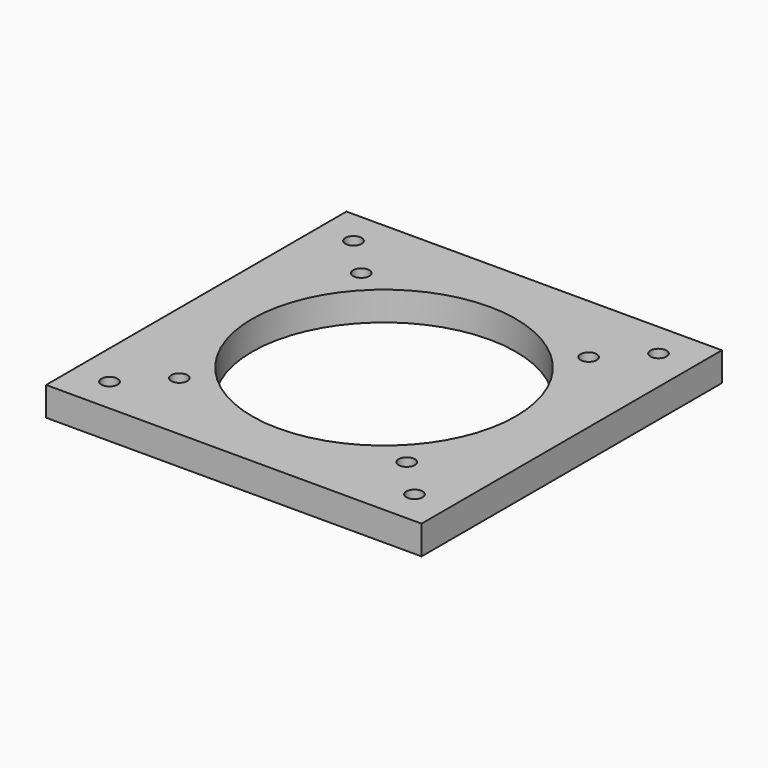
from build123d import *

# Parameters (mm, degrees)
F0_W     = 82.55
F0_H     = 82.55
F0_R     = 1.778
F0_R_2   = 28.9941
F1_DEPTH = 6.35


# Not quite as in the source:
# - a length typed as a fraction of an inch, garbled in the dataset ("3 / 203.2 mm" for 3/8 in), is restored


with BuildPart() as f1:
    # F0 (on Top) → F1 (new body)
    with BuildSketch(Plane.XY):
        Rectangle(F0_W, F0_H)
        with Locations((-33.528, -33.528)):
            Circle(F0_R, mode=Mode.SUBTRACT)
        with Locations((-24.9936, -24.9936)):
            Circle(F0_R, mode=Mode.SUBTRACT)
        with Locations((33.528, -33.528)):
            Circle(F0_R, mode=Mode.SUBTRACT)
        with Locations((24.9936, -24.9936)):
            Circle(F0_R, mode=Mode.SUBTRACT)
        with Locations((-24.9936, 24.9936)):
            Circle(F0_R, mode=Mode.SUBTRACT)
        with Locations((-33.528, 33.528)):
            Circle(F0_R, mode=Mode.SUBTRACT)
        Circle(F0_R_2, mode=Mode.SUBTRACT)
        with Locations((24.9936, 24.9936)):
            Circle(F0_R, mode=Mode.SUBTRACT)
        with Locations((33.528, 33.528)):
            Circle(F0_R, mode=Mode.SUBTRACT)
    extrude(amount=F1_DEPTH)


solid = f1.part
